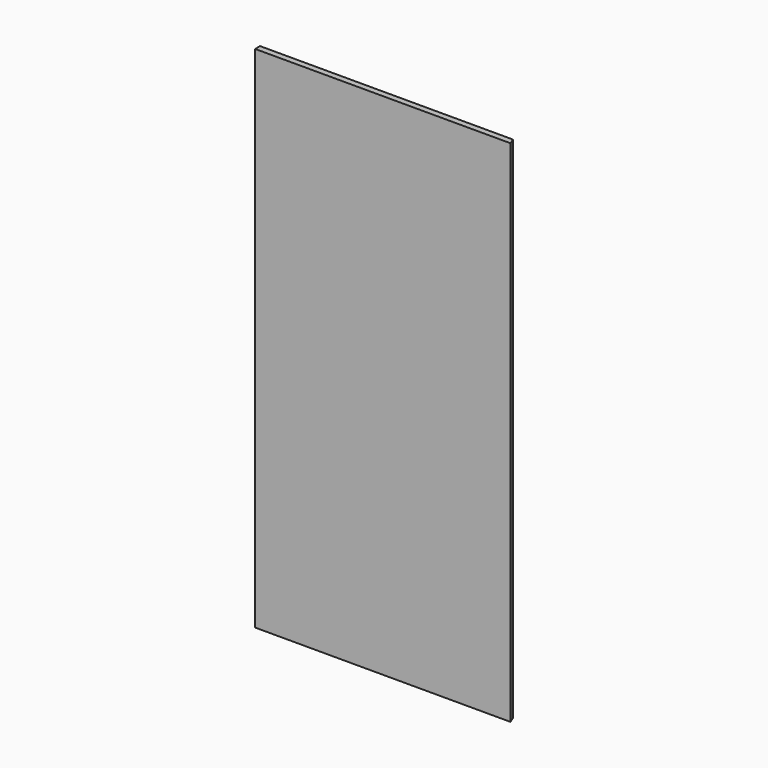
from build123d import *

# Parameters (mm, degrees)
F0_W     = 528.4471722421
F0_H     = 1054.1
F1_DEPTH = 12.7
F2_SIZE2 = 5.260502
F2_SIZE  = 12.69999


# Not quite as in the source:
# - a fillet or chamfer is up to 0.001 mm smaller than in the source, because OpenCascade refuses the exact size


with BuildPart() as f1:
    # F0 (on Front) → F1 (new body)
    with BuildSketch(Plane.XZ):
        with Locations((264.2235861211, 527.05)):
            Rectangle(F0_W, F0_H)
    extrude(amount=-F1_DEPTH)

    # F2 (size 12.7 and 5.2605122421 in the source; OpenCascade refuses exactly that, so slightly less here)
    f2_edges = [f1.edges().sort_by_distance(p)[0] for p in [
        (528.447172, 12.7, 527.05),
    ]]
    f2_side = f1.faces().sort_by_distance((528.447172, 6.35, 527.05))[0]
    chamfer(f2_edges, length=F2_SIZE, length2=F2_SIZE2, reference=f2_side)


solid = f1.part
